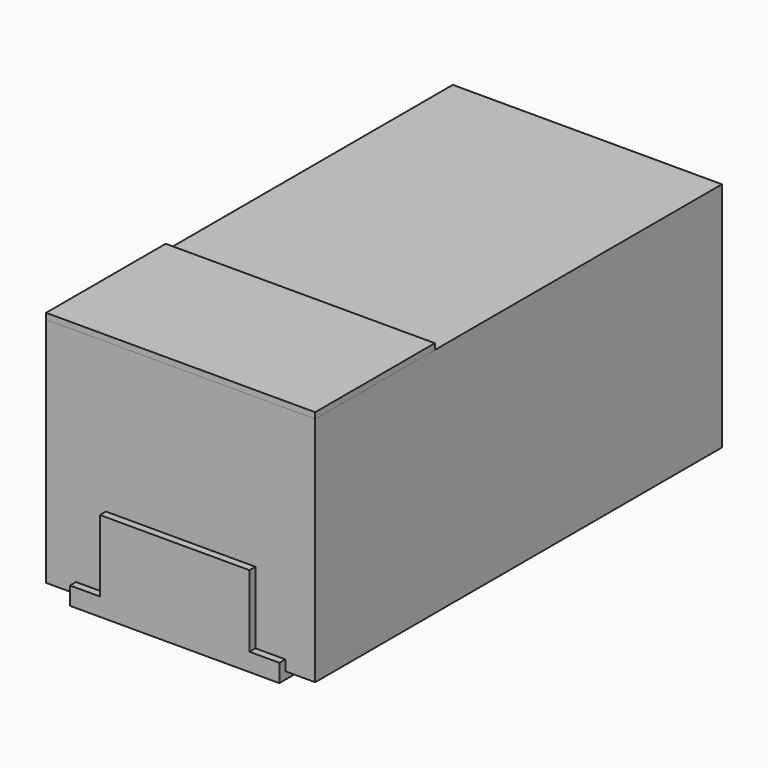
from build123d import *

# Parameters (mm, degrees)
F0_W          = 0.9
F0_H          = 1.7
F1_DEPTH      = 0.775
F2_W          = 0.9
F2_H          = 0.5
F3_DEPTH      = 0.02
F5_DEPTH      = 0.46
F7_DEPTH      = 0.876
F7_DEPTH_BACK = 0.876


with BuildPart() as f1:
    # F0 (on Top) → F1 (new body)
    with BuildSketch(Plane.XY):
        Rectangle(F0_W, F0_H)
    extrude(amount=F1_DEPTH)


with BuildPart() as f3:
    # F2 (on face) → F3 (new body)
    with BuildSketch(Plane.XY.offset(0.775)):
        with Locations((0, -0.6)):
            Rectangle(F2_W, F2_H)
    extrude(amount=F3_DEPTH)


with BuildPart() as f5:
    # F4 (on Right) → F5 (new body, symmetric)
    with BuildSketch(Plane.YZ):
        Polygon((-0.815, 0.035), (-0.815, 0.275), (-0.875, 0.275), (-0.875, -0.025), (-0.5, -0.025), (-0.5, 0.035), align=None)
    extrude(amount=F5_DEPTH, both=True)


with BuildPart() as f5b:
    # F4 (on Right) → F5, piece 2 (new body, symmetric)
    with BuildSketch(Plane.YZ):
        Polygon((0.875, 0.275), (0.815, 0.275), (0.815, 0.035), (0.5, 0.035), (0.5, -0.025), (0.875, -0.025), align=None)
    extrude(amount=F5_DEPTH, both=True)


with BuildPart() as f7_tool:
    # F6 (on Front) → F7 (new body, two sides)
    with BuildSketch(Plane.XZ) as f7_sk:
        Polygon((-0.25, 0.795), (-0.5751563585, 0.795), (-0.5751563585, -0.025), (-0.35, -0.025), (-0.35, 0.035), (-0.25, 0.035), align=None)
        Polygon((0.5751563585, -0.025), (0.5751563585, 0.795), (0.25, 0.795), (0.25, 0.035), (0.35, 0.035), (0.35, -0.025), align=None)
    extrude(amount=-F7_DEPTH)
    extrude(f7_sk.sketch, amount=F7_DEPTH_BACK)


with BuildPart() as f5_1:
    add(f5.part)

    # F7: cut by f7_tool
    add(f7_tool.part, mode=Mode.SUBTRACT)


with BuildPart() as f5b_1:
    add(f5b.part)

    # F7: cut by f7_tool
    add(f7_tool.part, mode=Mode.SUBTRACT)


solid = Compound([f1.part, f3.part, f5_1.part, f5b_1.part])
